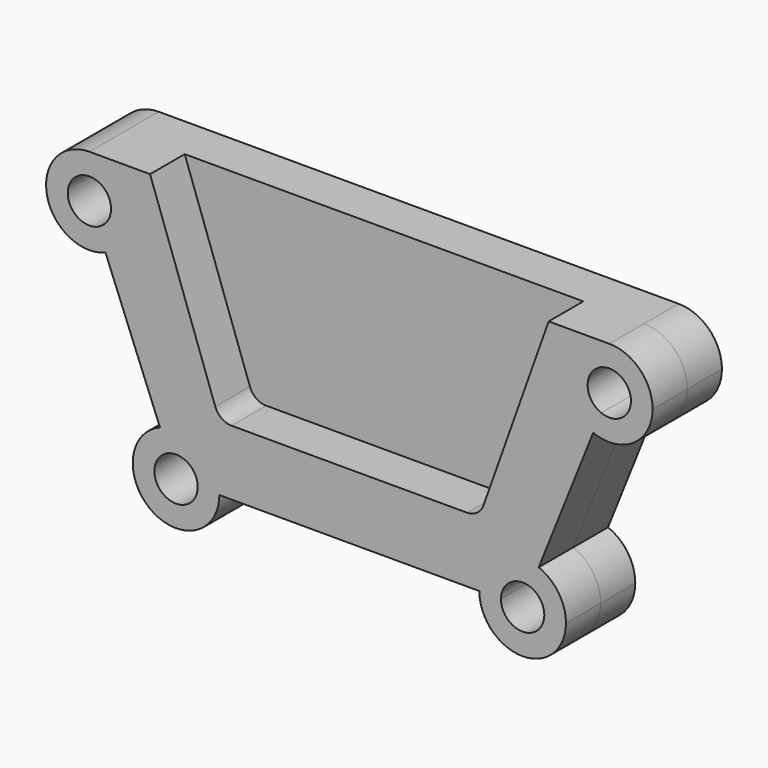
from build123d import *

# Parameters (mm, degrees)
F1_DEPTH = 12.7
F3_DEPTH = 38.1
F4_R     = 5.08


# Not quite as in the source:
# - a feature of the source that left no trace in its solid (it failed there, or was rolled back) is left out


with BuildPart() as f1:
    # F0 (on Front) → F1 (new body, symmetric)
    with BuildSketch(Plane.XZ):
        with BuildLine():
            Line((-38.1, -38.1), (0, -38.1))
            Line((0, -38.1), (38.1, -38.1))
            ThreePointArc((38.1, -38.1), (43.6800141218, -27.583546173), (55.5166615897, -26.3083460258))
            Line((55.5166615897, -26.3083460258), (71.4833384103, 13.6083460258))
            ThreePointArc((71.4833384103, 13.6083460258), (63.7291538885, 27.8016655187), (76.2, 38.1))
            Line((76.2, 38.1), (0, 38.1))
            Line((0, 38.1), (-76.2, 38.1))
            ThreePointArc((-76.2, 38.1), (-67.2197438789, 34.3802561211), (-63.5, 25.4))
            ThreePointArc((-63.5, 25.4), (-65.683546173, 18.2800141218), (-71.4833384103, 13.6083460258))
            Line((-71.4833384103, 13.6083460258), (-55.5166615897, -26.3083460258))
            ThreePointArc((-55.5166615897, -26.3083460258), (-43.6800141218, -27.583546173), (-38.1, -38.1))
        make_face()
        with BuildLine():
            ThreePointArc((55.5166615897, -26.3083460258), (43.6800141218, -27.583546173), (38.1, -38.1))
            Line((38.1, -38.1), (44.45, -38.1))
            ThreePointArc((44.45, -38.1), (47.2400070609, -32.8417730865), (53.1583307948, -32.2041730129))
            Line((53.1583307948, -32.2041730129), (55.5166615897, -26.3083460258))
        make_face()
        with BuildLine():
            Line((-44.45, -38.1), (-38.1, -38.1))
            ThreePointArc((-38.1, -38.1), (-43.6800141218, -27.583546173), (-55.5166615897, -26.3083460258))
            Line((-55.5166615897, -26.3083460258), (-53.1583307948, -32.2041730129))
            ThreePointArc((-53.1583307948, -32.2041730129), (-47.2400070609, -32.8417730865), (-44.45, -38.1))
        make_face()
        with BuildLine():
            ThreePointArc((-76.2, 38.1), (-88.6708461115, 22.9983344813), (-71.4833384103, 13.6083460258))
            ThreePointArc((-71.4833384103, 13.6083460258), (-65.683546173, 18.2800141218), (-63.5, 25.4))
            ThreePointArc((-63.5, 25.4), (-67.2197438789, 34.3802561211), (-76.2, 38.1))
        make_face()
        with BuildLine():
            ThreePointArc((-69.85, 25.4), (-70.9417730865, 21.8400070609), (-73.8416692052, 19.5041730129))
            ThreePointArc((-73.8416692052, 19.5041730129), (-81.4582269135, 28.9599929391), (-69.85, 25.4))
        make_face(mode=Mode.SUBTRACT)
        with BuildLine():
            ThreePointArc((76.2, 38.1), (63.7291538885, 27.8016655187), (71.4833384103, 13.6083460258))
            ThreePointArc((71.4833384103, 13.6083460258), (83.3199858782, 14.883546173), (88.9, 25.4))
            ThreePointArc((88.9, 25.4), (85.1802561211, 34.3802561211), (76.2, 38.1))
        make_face()
        with BuildLine():
            ThreePointArc((82.55, 25.4), (79.7599929391, 20.1417730865), (73.8416692052, 19.5041730129))
            ThreePointArc((73.8416692052, 19.5041730129), (72.6400070609, 30.6582269135), (82.55, 25.4))
        make_face(mode=Mode.SUBTRACT)
        with BuildLine():
            ThreePointArc((-55.5166615897, -26.3083460258), (-57.9199858782, -48.616453827), (-38.1, -38.1))
            Line((-38.1, -38.1), (-44.45, -38.1))
            ThreePointArc((-44.45, -38.1), (-54.3599929391, -43.3582269135), (-53.1583307948, -32.2041730129))
            Line((-53.1583307948, -32.2041730129), (-55.5166615897, -26.3083460258))
        make_face()
        with BuildLine():
            Line((44.45, -38.1), (38.1, -38.1))
            ThreePointArc((38.1, -38.1), (50.8, -50.8), (63.5, -38.1))
            ThreePointArc((63.5, -38.1), (61.316453827, -30.9800141218), (55.5166615897, -26.3083460258))
            Line((55.5166615897, -26.3083460258), (53.1583307948, -32.2041730129))
            ThreePointArc((53.1583307948, -32.2041730129), (56.0582269135, -34.5400070609), (57.15, -38.1))
            ThreePointArc((57.15, -38.1), (50.8, -44.45), (44.45, -38.1))
        make_face()
    extrude(amount=F1_DEPTH, both=True)

    # F2 (on Front) → F3 (cut)
    with BuildSketch(Plane.XZ):
        Polygon((-38.1, -19.05), (0, -19.05), (38.1, -19.05), (58.42, 38.1), (0, 38.1), (-58.42, 38.1), align=None)
    extrude(amount=F3_DEPTH, mode=Mode.SUBTRACT)

    # F4
    f4_edges = [f1.edges().sort_by_distance(p)[0] for p in [
        (-38.1, -6.35, -19.05),
        (38.1, -6.35, -19.05),
    ]]
    fillet(f4_edges, radius=F4_R)


solid = f1.part
